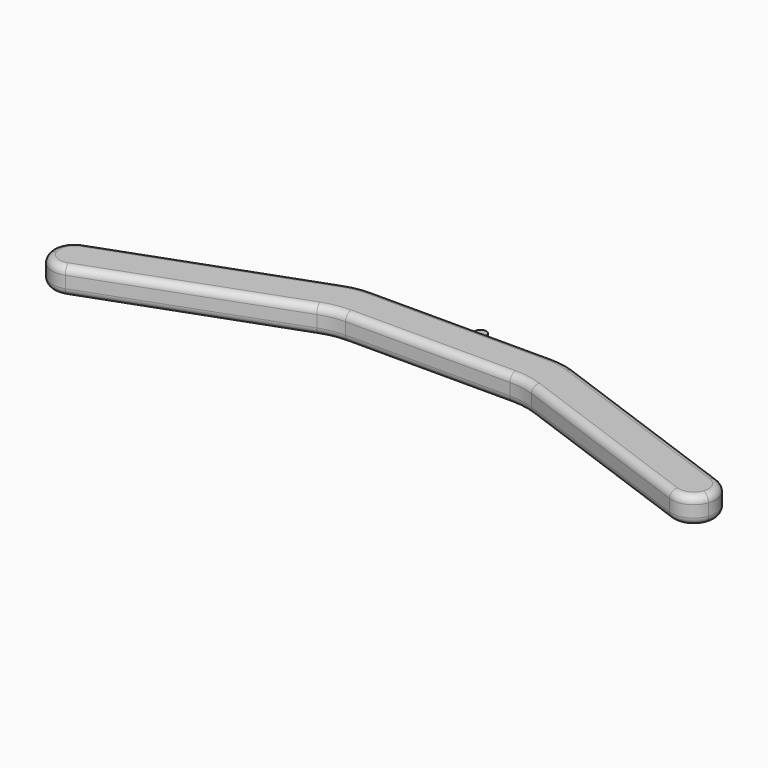
from build123d import *

# Parameters (mm, degrees)
F1_DEPTH = 18
F2_R     = 4
F3_DEPTH = 6
F4_R     = 4
F5_DEPTH = 6
F6_R     = 4.99999


# Not quite as in the source:
# - a fillet or chamfer is up to 0.001 mm smaller than in the source, because OpenCascade refuses the exact size


with BuildPart() as f1:
    # F0 (on Top) → F1 (new body)
    with BuildSketch(Plane.XY):
        with BuildLine():
            Line((61.1836509646, 0), (0, 0))
            Line((0, 0), (-61.1836509646, 0))
            ThreePointArc((-61.1836509646, 0), (-69.8660598479, -0.7596123494), (-78.2846581309, -3.0153689607))
            Line((-78.2846581309, -3.0153689607), (-215.6523562218, -53.0131222155))
            ThreePointArc((-215.6523562218, -53.0131222155), (-224.1166708775, -60.7692376012), (-224.6174433837, -72.2388136772))
            ThreePointArc((-224.6174433837, -72.2388136772), (-216.861327998, -80.7031283328), (-205.391751922, -81.2039008391))
            Line((-205.391751922, -81.2039008391), (-72.9948487096, -33.0153689607))
            ThreePointArc((-72.9948487096, -33.0153689607), (-64.5762504267, -30.7596123494), (-55.8938415433, -30))
            Line((-55.8938415433, -30), (0, -30))
            Line((0, -30), (55.8938415433, -30))
            ThreePointArc((55.8938415433, -30), (64.5762504267, -30.7596123494), (72.9948487096, -33.0153689607))
            Line((72.9948487096, -33.0153689607), (205.391751922, -81.2039008391))
            ThreePointArc((205.391751922, -81.2039008391), (216.861327998, -80.7031283328), (224.6174433837, -72.2388136772))
            ThreePointArc((224.6174433837, -72.2388136772), (224.1166708775, -60.7692376012), (215.6523562218, -53.0131222155))
            Line((215.6523562218, -53.0131222155), (78.2846581309, -3.0153689607))
            ThreePointArc((78.2846581309, -3.0153689607), (69.8660598479, -0.7596123494), (61.1836509646, 0))
        make_face()
    extrude(amount=F1_DEPTH)

    # F2 (on face) → F3 (cut)
    with BuildSketch(Plane(origin=(0, 0, 0), x_dir=(-1, 0, 0), z_dir=(0, 1, 0))):
        with Locations((0, 9)):
            Circle(F2_R)
    extrude(amount=-F3_DEPTH, mode=Mode.SUBTRACT)

    # F6 (radius 5 in the source; OpenCascade refuses exactly that, so slightly less here)
    f6_edges = [f1.edges().sort_by_distance(p)[0] for p in [
        (0, 0, 0),
        (0, 0, 18),
    ]]
    fillet(f6_edges, radius=F6_R)


with BuildPart() as f5:
    # F4 (on Top) → F5 (new body)
    with BuildSketch(Plane.XY):
        with Locations((0, 14.8481540382)):
            Circle(F4_R)
    extrude(amount=F5_DEPTH)


solid = Compound([f1.part, f5.part])
